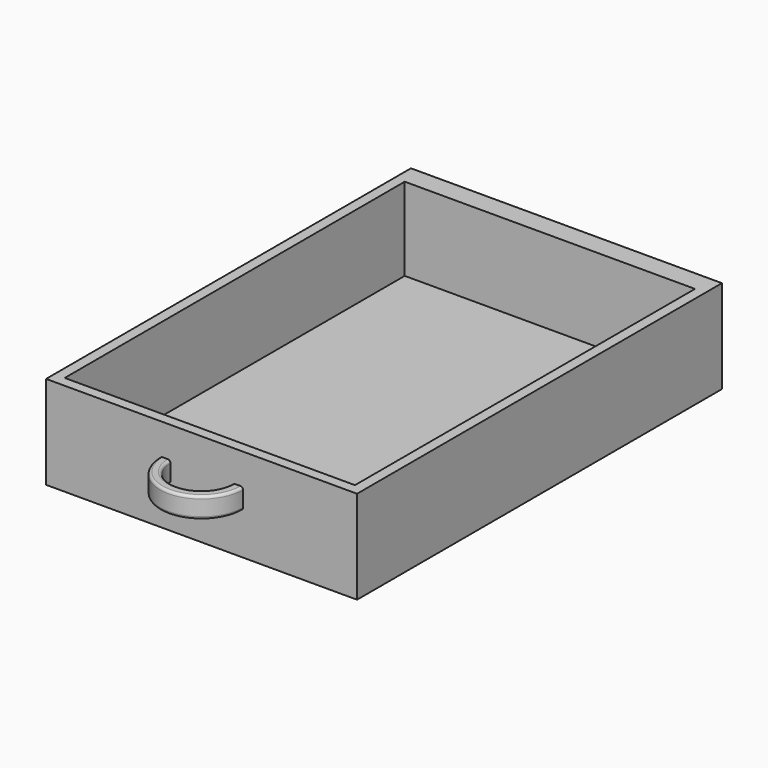
from build123d import *

# Parameters (mm, degrees)
F0_W     = 381
F0_H     = 114.3
F1_DEPTH = 558.8
F2_W     = 355.6
F2_H     = 520.7
F3_DEPTH = 101.6
F4_W     = 50.8
F4_H     = 12.7
F5_ANGLE = 180
F7_DEPTH = 76.201
F8_R     = 3.175


# Not quite as in the source:
# - a feature names something its author has since deleted; it is built from what else it names


with BuildPart() as f1:
    # F0 (on Front) → F1 (new body)
    with BuildSketch(Plane.XZ):
        with Locations((157.0888143581, 38.9549015626)):
            Rectangle(F0_W, F0_H)
    extrude(amount=-F1_DEPTH)

    # F2 (on face) → F3 (cut)
    with BuildSketch(Plane.XY.offset(96.1049015626)):
        with Locations((157.0888143581, 273.05)):
            Rectangle(F2_W, F2_H)
    extrude(amount=-F3_DEPTH, mode=Mode.SUBTRACT)

    # F4 (on face) → F5 (revolve)
    with BuildSketch(Plane.XZ):
        with Locations((131.6888143581, 51.6549015626)):
            Rectangle(F4_W, F4_H)
        with Locations((131.6888143581, 38.9549015626)):
            Rectangle(F4_W, F4_H)
    revolve(axis=Axis((157.0888143581, 0, 45.3049015626), (0, 0, 1)), revolution_arc=F5_ANGLE)

    # F6 (on face) → F7 (cut, through all)
    with BuildSketch(Plane.XY.offset(58.0049015626)):
        with BuildLine():
            Line((195.1888143581, 0), (118.9888143581, 0))
            ThreePointArc((118.9888143581, 0), (157.0888143581, -38.1), (195.1888143581, 0))
        make_face()
    extrude(amount=-F7_DEPTH, mode=Mode.SUBTRACT)

    # F8
    f8_edges = [f1.edges().sort_by_distance(p)[0] for p in [
        (157.088814, -50.8, 58.004902),
        (157.088814, -38.1, 58.004902),
        (157.088814, -50.8, 32.604902),
        (157.088814, -38.1, 32.604902),
    ]]
    fillet(f8_edges, radius=F8_R)


solid = f1.part
